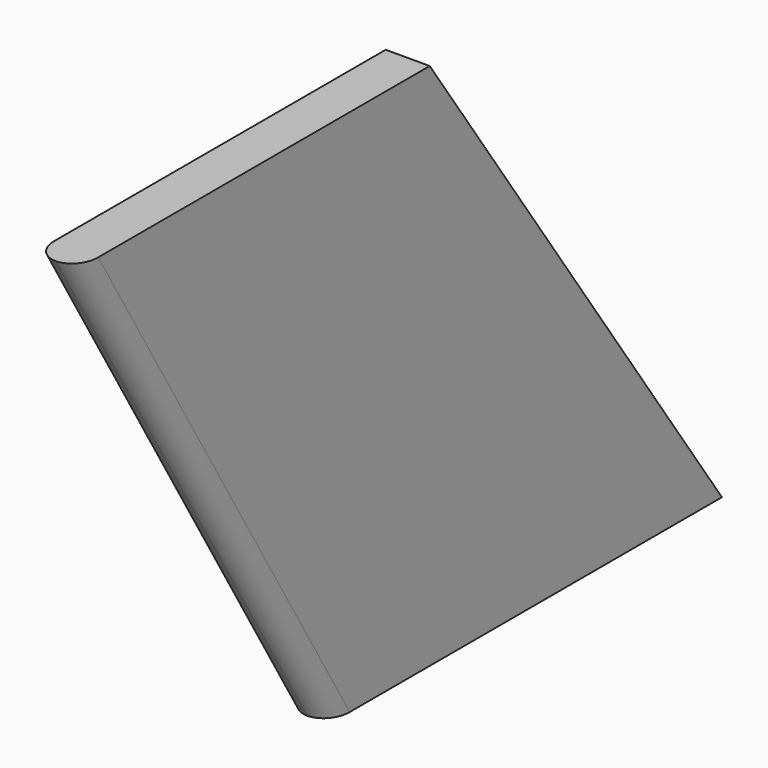
from build123d import *

# Parameters (mm, degrees)
F1_DEPTH = 10
F2_R     = 4.99999


# Not quite as in the source:
# - a fillet or chamfer is up to 0.001 mm smaller than in the source, because OpenCascade refuses the exact size


with BuildPart() as f1:
    # F0 (on Right) → F1 (new body)
    with BuildSketch(Plane.YZ):
        Polygon((0, 120), (0, 0), (111.5350200628, 0), (28.5433451417, 120), align=None)
        Polygon((-71.4566548583, 120), (0, 0), (0, 120), align=None)
    extrude(amount=F1_DEPTH)

    # F2 (radius 5 in the source; OpenCascade refuses exactly that, so slightly less here)
    f2_edges = [f1.edges().sort_by_distance(p)[0] for p in [
        (0, -35.728327, 60),
        (10, -35.728327, 60),
    ]]
    fillet(f2_edges, radius=F2_R)


solid = f1.part
